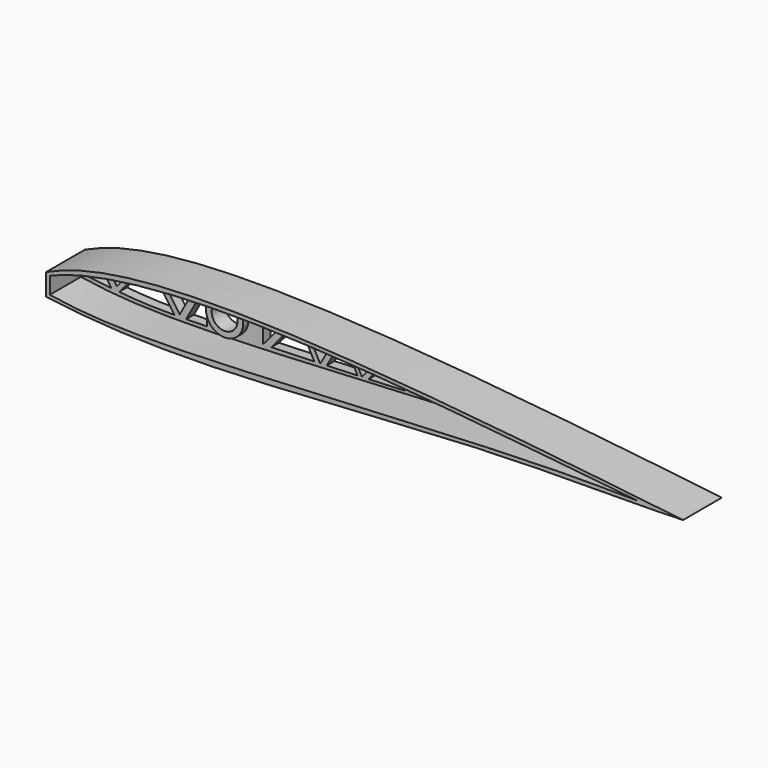
from build123d import *

# Parameters (mm, degrees)
F0_R     = 5.75
F0_R_2   = 2.5
F1_DEPTH = 3
F2_DEPTH = 15
F0_R_3   = 4
F3_DEPTH = 5


# Not quite as in the source:
# - ends of sketch curves that miss each other by under 0.0002 mm in the source are joined


with BuildPart() as f1:
    # F0 (on Front) → F1 (new body)
    with BuildSketch(Plane.XZ):
        with BuildLine():
            add(Edge.make_bspline(
                [(-96.5428803444, -1.7252441192), (-96.4749771743, -1.6951094214), (-96.406839482, -1.6654244391), (-96.3385477662, -1.6362179573)],
                knots=[0.9799990925, 0.9799990925, 0.9799990925, 0.9799990925, 1, 1, 1, 1], degree=3))
            Line((-96.5428803444, -1.7252441192), (-96.5428803444, -6.1999121678))
            add(Edge.make_bspline(
                [(-96.5428803445, -6.1999121678), (-96.1611087474, -6.2678718719), (-95.7782117135, -6.3340115071), (-95.3941463942, -6.3983665862)],
                knots=[0.0058166358, 0.0058166358, 0.0058166358, 0.0058166358, 0.0137332718, 0.0137332718, 0.0137332718, 0.0137332718], degree=3))
            Line((-95.3941463942, -6.3983665862), (-95.3941463942, -1.2117682704))
            add(Edge.make_bspline(
                [(-96.3385477662, -1.6362179573), (-96.0300606253, -1.4927727074), (-95.71523374, -1.3512900387), (-95.3941463942, -1.2117682704)],
                knots=[0, 0, 0, 0, 0.0112083174, 0.0112083174, 0.0112083174, 0.0112083174], degree=3))
        make_face()
        with BuildLine():
            Line((-95.3941463942, -1.2117682704), (-95.3941463942, -6.3983665862))
            add(Edge.make_bspline(
                [(-95.3941463942, -6.3983665862), (-80.8694306992, -8.8321693274), (-43.0853796331, -8.5556683111), (40.9195716837, -3.3120714751), (72.7341022162, -3.1550192186), (86.094097513, -3.3751911245)],
                knots=[0.0137332718, 0.0137332718, 0.0137332718, 0.0137332718, 0.3131273629, 0.7122131732, 1, 1, 1, 1], degree=3))
            add(Edge.make_bspline(
                [(-95.3941463942, -1.2117682704), (-84.6882492469, 3.4402546795), (-37.9471480513, 9.9808619504), (36.943279708, 1.696590452), (86.094097513, -3.3751911245)],
                knots=[0.0112083174, 0.0112083174, 0.0112083174, 0.0112083174, 0.384923117, 1, 1, 1, 1], degree=3))
        make_face()
        with BuildLine():
            add(Edge.make_bspline(
                [(-58.7596564737, 4.4301702308), (-57.9753522042, 4.4434334419), (-57.1958768535, 4.4485089516), (-56.4223485914, 4.4453240584)],
                knots=[0.9373807911, 0.9373807911, 0.9373807911, 0.9373807911, 1, 1, 1, 1], degree=3))
            Line((-56.4223485914, 4.4453240584), (-56.4223485914, -7.2081234653))
            add(Edge.make_bspline(
                [(-56.4223485914, -7.2081234653), (-58.5959136423, -7.2589059214), (-60.7694786933, -7.3096883775), (-62.937808184, -7.3435649348)],
                knots=[0, 0, 0, 0, 0.1686137564, 0.1686137564, 0.1686137564, 0.1686137564], degree=3))
            add(Edge.make_bspline(
                [(-62.937808184, -7.3435649348), (-64.1162804896, -7.3619766129), (-65.2932062899, -7.3753945447), (-66.4677450702, -7.3811046631)],
                knots=[0.1686137564, 0.1686137564, 0.1686137564, 0.1686137564, 0.2602541842, 0.2602541842, 0.2602541842, 0.2602541842], degree=3))
            add(Edge.make_bspline(
                [(-66.4677450702, -7.3811046631), (-69.6195281104, -7.3964273197), (-75.381287574, -7.3225727781), (-81.0300999392, -6.8840061254), (-83.592082751, -6.6398550354)],
                knots=[0.2602541842, 0.2602541842, 0.2602541842, 0.2602541842, 0.5061641117, 0.7122660034, 0.7122660034, 0.7122660034, 0.7122660034], degree=3))
            add(Edge.make_bspline(
                [(-83.592082751, -6.6398550354), (-84.4022359708, -6.5626492904), (-85.2110210526, -6.4810257561), (-86.0187478894, -6.3959850932)],
                knots=[0.7122660034, 0.7122660034, 0.7122660034, 0.7122660034, 0.7774397861, 0.7774397861, 0.7774397861, 0.7774397861], degree=3))
            add(Edge.make_bspline(
                [(-86.0187478894, -6.3959850932), (-88.7770327399, -6.1055819993), (-91.5229770142, -5.7753305369), (-94.2689212885, -5.4450790744)],
                knots=[0.7774397861, 0.7774397861, 0.7774397861, 0.7774397861, 1, 1, 1, 1], degree=3))
            Line((-94.2689212885, -5.4450790744), (-94.2689212885, -1.6795024276))
            add(Edge.make_bspline(
                [(-94.2689212885, -1.6795024276), (-92.8628953972, -1.1841994891), (-91.4581917851, -0.7250541475), (-90.0523380192, -0.2995832154)],
                knots=[0, 0, 0, 0, 0.113305349, 0.113305349, 0.113305349, 0.113305349], degree=3))
            add(Edge.make_bspline(
                [(-90.0523380192, -0.2995832154), (-89.3811327558, -0.0964480559), (-88.7096653203, 0.0990111844), (-88.0376666398, 0.2870647488)],
                knots=[0.113305349, 0.113305349, 0.113305349, 0.113305349, 0.1674014069, 0.1674014069, 0.1674014069, 0.1674014069], degree=3))
            add(Edge.make_bspline(
                [(-88.0376666398, 0.2870647488), (-84.5719605974, 1.2569154246), (-81.0921245769, 2.0297910107), (-77.561248917, 2.6427617143)],
                knots=[0.1674014069, 0.1674014069, 0.1674014069, 0.1674014069, 0.4463915894, 0.4463915894, 0.4463915894, 0.4463915894], degree=3))
            add(Edge.make_bspline(
                [(-77.561248917, 2.6427617143), (-76.8555880554, 2.7652665761), (-76.1478885806, 2.8813845552), (-75.4378558602, 2.991411566)],
                knots=[0.4463915894, 0.4463915894, 0.4463915894, 0.4463915894, 0.5021489911, 0.5021489911, 0.5021489911, 0.5021489911], degree=3))
            add(Edge.make_bspline(
                [(-75.4378558602, 2.991411566), (-74.9289069597, 3.0702785315), (-74.4187592444, 3.1460159753), (-73.9077034377, 3.2186049948)],
                knots=[0.5021489911, 0.5021489911, 0.5021489911, 0.5021489911, 0.5421156961, 0.5421156961, 0.5421156961, 0.5421156961], degree=3))
            add(Edge.make_bspline(
                [(-73.9077034377, 3.2186049948), (-73.2834974958, 3.3072655612), (-72.6579368364, 3.3912292161), (-72.0315511948, 3.4704615167)],
                knots=[0.5421156961, 0.5421156961, 0.5421156961, 0.5421156961, 0.5909312157, 0.5909312157, 0.5909312157, 0.5909312157], degree=3))
            add(Edge.make_bspline(
                [(-72.0315511948, 3.4704615167), (-67.5860174529, 4.0327826216), (-63.0989300921, 4.3567896513), (-58.7596564737, 4.4301702308)],
                knots=[0.5909312157, 0.5909312157, 0.5909312157, 0.5909312157, 0.9373807911, 0.9373807911, 0.9373807911, 0.9373807911], degree=3))
        make_face(mode=Mode.SUBTRACT)
        with Locations((-49.452, -1.371)):
            Circle(F0_R, mode=Mode.SUBTRACT)
        with BuildLine():
            Line((-39.2314642668, -6.5102223307), (-39.2314642668, 5.299675744))
            add(Edge.make_bspline(
                [(-39.2314642668, 5.299675744), (-35.9534074438, 5.1909875249), (-32.6753506208, 5.0822993057), (-29.3931825657, 4.965637255)],
                knots=[0, 0, 0, 0, 0.1482033118, 0.1482033118, 0.1482033118, 0.1482033118], degree=3))
            add(Edge.make_bspline(
                [(-29.3931825657, 4.965637255), (-28.6917369238, 4.940704928), (-27.9901035066, 4.9154084065), (-27.2882421839, 4.8896698568)],
                knots=[0.1482033118, 0.1482033118, 0.1482033118, 0.1482033118, 0.1798764515, 0.1798764515, 0.1798764515, 0.1798764515], degree=3))
            add(Edge.make_bspline(
                [(-27.2882421839, 4.8896698568), (-23.4137483209, 4.7475850185), (-19.5323092994, 4.5920298819), (-15.6371742048, 4.4099108889)],
                knots=[0.1798764515, 0.1798764515, 0.1798764515, 0.1798764515, 0.3547220816, 0.3547220816, 0.3547220816, 0.3547220816], degree=3))
            add(Edge.make_bspline(
                [(-15.6371742048, 4.4099108889), (-15.0215280405, 4.3811260441), (-14.4055397287, 4.3516775961), (-13.7891826138, 4.3215138457)],
                knots=[0.3547220816, 0.3547220816, 0.3547220816, 0.3547220816, 0.382357334, 0.382357334, 0.382357334, 0.382357334], degree=3))
            add(Edge.make_bspline(
                [(-13.7891826138, 4.3215138457), (-11.2804707946, 4.1987406107), (-7.2510801006, 3.9830392372), (-3.2013896807, 3.7279660672), (-1.676706941, 3.6272723386)],
                knots=[0.382357334, 0.382357334, 0.382357334, 0.382357334, 0.4948390149, 0.5625818971, 0.5625818971, 0.5625818971, 0.5625818971], degree=3))
            add(Edge.make_bspline(
                [(-1.676706941, 3.6272723386), (-1.1181316432, 3.5903826775), (-0.5592230256, 3.552846535), (0, 3.5147005908)],
                knots=[0.5625818971, 0.5625818971, 0.5625818971, 0.5625818971, 0.5873998474, 0.5873998474, 0.5873998474, 0.5873998474], degree=3))
            add(Edge.make_bspline(
                [(0, 3.5147005908), (3.5849822281, 3.2701603521), (7.1828854983, 3.000559448), (10.7887274401, 2.7155613037)],
                knots=[0.5873998474, 0.5873998474, 0.5873998474, 0.5873998474, 0.7464990028, 0.7464990028, 0.7464990028, 0.7464990028], degree=3))
            add(Edge.make_bspline(
                [(10.7887274401, 2.7155613037), (11.5803406425, 2.6529938652), (12.3723364586, 2.5896843385), (13.1646621709, 2.5257349704)],
                knots=[0.7464990028, 0.7464990028, 0.7464990028, 0.7464990028, 0.7814270428, 0.7814270428, 0.7814270428, 0.7814270428], degree=3))
            add(Edge.make_bspline(
                [(13.1646621709, 2.5257349704), (15.5409627422, 2.3339414724), (17.9202306891, 2.1363926795), (20.3010438532, 1.9358469013)],
                knots=[0.7814270428, 0.7814270428, 0.7814270428, 0.7814270428, 0.8861813381, 0.8861813381, 0.8861813381, 0.8861813381], degree=3))
            add(Edge.make_bspline(
                [(20.3010438532, 1.9358469013), (21.4384423664, 1.8400391019), (22.5761935461, 1.7435472975), (23.7141423287, 1.6466722377)],
                knots=[0.8861813381, 0.8861813381, 0.8861813381, 0.8861813381, 0.9362261637, 0.9362261637, 0.9362261637, 0.9362261637], degree=3))
            add(Edge.make_bspline(
                [(23.7141423287, 1.6466722377), (25.1642694588, 1.523221029), (26.6147174818, 1.3991474412), (28.0651655048, 1.2750738533)],
                knots=[0.9362261637, 0.9362261637, 0.9362261637, 0.9362261637, 1, 1, 1, 1], degree=3))
            Line((28.0651655048, 1.2750738533), (28.0651655048, -3.6732077133))
            add(Edge.make_bspline(
                [(28.0651655048, -3.6732077133), (27.4664662691, -3.7032045951), (26.8677670333, -3.7332014769), (26.269106513, -3.7631839579)],
                knots=[0, 0, 0, 0, 0.0260461999, 0.0260461999, 0.0260461999, 0.0260461999], degree=3))
            add(Edge.make_bspline(
                [(26.269106513, -3.7631839579), (23.6217461688, -3.8957706721), (20.9751429176, -4.0280757752), (18.3326447297, -4.1588539429)],
                knots=[0.0260461999, 0.0260461999, 0.0260461999, 0.0260461999, 0.1412261299, 0.1412261299, 0.1412261299, 0.1412261299], degree=3))
            add(Edge.make_bspline(
                [(18.3326447297, -4.1588539429), (17.592409558, -4.1954884427), (16.8524965153, -4.2320031222), (16.1129791965, -4.2683706067)],
                knots=[0.1412261299, 0.1412261299, 0.1412261299, 0.1412261299, 0.1734911417, 0.1734911417, 0.1734911417, 0.1734911417], degree=3))
            add(Edge.make_bspline(
                [(16.1129791965, -4.2683706067), (15.6061303016, -4.2932960802), (15.0994672951, -4.3181524099), (14.5930138711, -4.3429307826)],
                knots=[0.1734911417, 0.1734911417, 0.1734911417, 0.1734911417, 0.1956048707, 0.1956048707, 0.1956048707, 0.1956048707], degree=3))
            add(Edge.make_bspline(
                [(14.5930138711, -4.3429307826), (12.3936169659, -4.4505368792), (10.1981726621, -4.5566727509), (8.0086215303, -4.6606165755)],
                knots=[0.1956048707, 0.1956048707, 0.1956048707, 0.1956048707, 0.2916391057, 0.2916391057, 0.2916391057, 0.2916391057], degree=3))
            add(Edge.make_bspline(
                [(8.0086215303, -4.6606165755), (7.3735996711, -4.6907627547), (6.739073509, -4.7207245525), (6.105090384, -4.7504843601)],
                knots=[0.2916391057, 0.2916391057, 0.2916391057, 0.2916391057, 0.3194913159, 0.3194913159, 0.3194913159, 0.3194913159], degree=3))
            add(Edge.make_bspline(
                [(6.105090384, -4.7504843601), (5.6209562477, -4.773210105), (5.1371387803, -4.7958180605), (4.6536590632, -4.818300385)],
                knots=[0.3194913159, 0.3194913159, 0.3194913159, 0.3194913159, 0.3407603453, 0.3407603453, 0.3407603453, 0.3407603453], degree=3))
            add(Edge.make_bspline(
                [(4.6536590632, -4.818300385), (0.8798372036, -4.9937871426), (-2.8734067176, -5.1616196506), (-6.5960472566, -5.3180688061)],
                knots=[0.3407603453, 0.3407603453, 0.3407603453, 0.3407603453, 0.5067766752, 0.5067766752, 0.5067766752, 0.5067766752], degree=3))
            add(Edge.make_bspline(
                [(-6.5960472566, -5.3180688061), (-6.6322875139, -5.3195918534), (-7.325510614, -5.3487072139), (-8.0176689199, -5.3774265095), (-8.6727461513, -5.4043100041)],
                knots=[0.5067766752, 0.5067766752, 0.5067766752, 0.5067766752, 0.5083928599, 0.5376943974, 0.5376943974, 0.5376943974, 0.5376943974], degree=3))
            add(Edge.make_bspline(
                [(-8.6727461513, -5.4043100041), (-9.1152981748, -5.422471748), (-9.557439724, -5.4404808103), (-9.9991883747, -5.4583437286)],
                knots=[0.5376943974, 0.5376943974, 0.5376943974, 0.5376943974, 0.5574897042, 0.5574897042, 0.5574897042, 0.5574897042], degree=3))
            add(Edge.make_bspline(
                [(-9.9991883747, -5.4583437286), (-13.1995651312, -5.5877568424), (-16.3793198272, -5.7094992948), (-19.5451358525, -5.8260570653)],
                knots=[0.5574897042, 0.5574897042, 0.5574897042, 0.5574897042, 0.7009025691, 0.7009025691, 0.7009025691, 0.7009025691], degree=3))
            add(Edge.make_bspline(
                [(-19.5451358525, -5.8260570653), (-20.1920530868, -5.8498750098), (-20.8383882883, -5.8734764592), (-21.4841984848, -5.8968826257)],
                knots=[0.7009025691, 0.7009025691, 0.7009025691, 0.7009025691, 0.7302082057, 0.7302082057, 0.7302082057, 0.7302082057], degree=3))
            add(Edge.make_bspline(
                [(-21.4841984848, -5.8968826257), (-21.5265905055, -5.8984190441), (-21.568980264, -5.8999546211), (-21.6113677766, -5.9014893627)],
                knots=[0.7302082057, 0.7302082057, 0.7302082057, 0.7302082057, 0.7321318749, 0.7321318749, 0.7321318749, 0.7321318749], degree=3))
            add(Edge.make_bspline(
                [(-21.6113677766, -5.9014893627), (-22.2032423382, -5.9229196008), (-22.7946789769, -5.9441869474), (-23.3857216062, -5.9653077367)],
                knots=[0.7321318749, 0.7321318749, 0.7321318749, 0.7321318749, 0.7589928716, 0.7589928716, 0.7589928716, 0.7589928716], degree=3))
            add(Edge.make_bspline(
                [(-23.3857216062, -5.9653077367), (-27.8246304727, -6.1239312512), (-32.2413153798, -6.2742882557), (-36.6543788181, -6.4232982046)],
                knots=[0.7589928716, 0.7589928716, 0.7589928716, 0.7589928716, 0.9607270796, 0.9607270796, 0.9607270796, 0.9607270796], degree=3))
            add(Edge.make_bspline(
                [(-36.6543788181, -6.4232982046), (-37.5134988009, -6.452306948), (-38.3724815339, -6.4812646393), (-39.2314642668, -6.5102223307)],
                knots=[0.9607270796, 0.9607270796, 0.9607270796, 0.9607270796, 1, 1, 1, 1], degree=3))
        make_face(mode=Mode.SUBTRACT)
        with Locations((33.779, -1.031)):
            Circle(F0_R_2, mode=Mode.SUBTRACT)
        with BuildLine():
            Line((-62.937808184, -7.3435649348), (-56.4223485914, 4.4453240584))
            add(Edge.make_bspline(
                [(-58.7596564737, 4.4301702308), (-57.9753522042, 4.4434334419), (-57.1958768535, 4.4485089516), (-56.4223485914, 4.4453240584)],
                knots=[0.9373807911, 0.9373807911, 0.9373807911, 0.9373807911, 1, 1, 1, 1], degree=3))
            Line((-58.7596564737, 4.4301702308), (-64.903050668, -6.6855141148))
            Line((-64.903050668, -6.6855141148), (-72.0315511948, 3.4704615167))
            add(Edge.make_bspline(
                [(-73.9077034377, 3.2186049948), (-73.2834974958, 3.3072655612), (-72.6579368364, 3.3912292161), (-72.0315511948, 3.4704615167)],
                knots=[0.5421156961, 0.5421156961, 0.5421156961, 0.5421156961, 0.5909312157, 0.5909312157, 0.5909312157, 0.5909312157], degree=3))
            Line((-73.9077034377, 3.2186049948), (-66.4677450702, -7.3811046631))
            add(Edge.make_bspline(
                [(-62.937808184, -7.3435649348), (-64.1162804896, -7.3619766129), (-65.2932062899, -7.3753945447), (-66.4677450702, -7.3811046631)],
                knots=[0.1686137564, 0.1686137564, 0.1686137564, 0.1686137564, 0.2602541842, 0.2602541842, 0.2602541842, 0.2602541842], degree=3))
        make_face()
        with BuildLine():
            add(Edge.make_bspline(
                [(-83.592082751, -6.6398550354), (-84.4022359708, -6.5626492904), (-85.2110210526, -6.4810257561), (-86.0187478894, -6.3959850932)],
                knots=[0.7122660034, 0.7122660034, 0.7122660034, 0.7122660034, 0.7774397861, 0.7774397861, 0.7774397861, 0.7774397861], degree=3))
            Line((-83.592082751, -6.6398550354), (-75.4378558602, 2.991411566))
            add(Edge.make_bspline(
                [(-77.561248917, 2.6427617143), (-76.8555880554, 2.7652665761), (-76.1478885806, 2.8813845552), (-75.4378558602, 2.991411566)],
                knots=[0.4463915894, 0.4463915894, 0.4463915894, 0.4463915894, 0.5021489911, 0.5021489911, 0.5021489911, 0.5021489911], degree=3))
            Line((-77.561248917, 2.6427617143), (-84.3168773909, -5.3365672599))
            Line((-84.3168773909, -5.3365672599), (-88.0376666398, 0.2870647488))
            add(Edge.make_bspline(
                [(-90.0523380192, -0.2995832154), (-89.3811327558, -0.0964480559), (-88.7096653203, 0.0990111844), (-88.0376666398, 0.2870647488)],
                knots=[0.113305349, 0.113305349, 0.113305349, 0.113305349, 0.1674014069, 0.1674014069, 0.1674014069, 0.1674014069], degree=3))
            Line((-90.0523380192, -0.2995832154), (-86.0187478894, -6.3959850932))
        make_face()
        with BuildLine():
            Line((-29.3931825657, 4.965637255), (-39.2314642668, -6.5102223307))
            add(Edge.make_bspline(
                [(-36.6543788181, -6.4232982046), (-37.5134988009, -6.452306948), (-38.3724815339, -6.4812646393), (-39.2314642668, -6.5102223307)],
                knots=[0.9607270796, 0.9607270796, 0.9607270796, 0.9607270796, 1, 1, 1, 1], degree=3))
            Line((-36.6543788181, -6.4232982046), (-28.2822091366, 3.3424156275))
            Line((-28.2822091366, 3.3424156275), (-23.3857216062, -5.9653077367))
            add(Edge.make_bspline(
                [(-21.6113677766, -5.9014893627), (-22.2032423382, -5.9229196008), (-22.7946789769, -5.9441869474), (-23.3857216062, -5.9653077367)],
                knots=[0.7321318749, 0.7321318749, 0.7321318749, 0.7321318749, 0.7589928716, 0.7589928716, 0.7589928716, 0.7589928716], degree=3))
            Line((-21.6113677766, -5.9014893627), (-27.2882421839, 4.8896698568))
            add(Edge.make_bspline(
                [(-29.3931825657, 4.965637255), (-28.6917369238, 4.940704928), (-27.9901035066, 4.9154084065), (-27.2882421839, 4.8896698568)],
                knots=[0.1482033118, 0.1482033118, 0.1482033118, 0.1482033118, 0.1798764515, 0.1798764515, 0.1798764515, 0.1798764515], degree=3))
        make_face()
        with BuildLine():
            add(Edge.make_bspline(
                [(-15.6371742048, 4.4099108889), (-15.0215280405, 4.3811260441), (-14.4055397287, 4.3516775961), (-13.7891826138, 4.3215138457)],
                knots=[0.3547220816, 0.3547220816, 0.3547220816, 0.3547220816, 0.382357334, 0.382357334, 0.382357334, 0.382357334], degree=3))
            Line((-15.6371742048, 4.4099108889), (-21.4841984848, -5.8968826257))
            add(Edge.make_bspline(
                [(-19.5451358525, -5.8260570653), (-20.1920530868, -5.8498750098), (-20.8383882883, -5.8734764592), (-21.4841984848, -5.8968826257)],
                knots=[0.7009025691, 0.7009025691, 0.7009025691, 0.7009025691, 0.7302082057, 0.7302082057, 0.7302082057, 0.7302082057], degree=3))
            Line((-19.5451358525, -5.8260570653), (-14.4918043747, 3.0816610505))
            Line((-14.4918043747, 3.0816610505), (-9.9991883747, -5.4583437286))
            add(Edge.make_bspline(
                [(-8.6727461513, -5.4043100041), (-9.1152981748, -5.422471748), (-9.557439724, -5.4404808103), (-9.9991883747, -5.4583437286)],
                knots=[0.5376943974, 0.5376943974, 0.5376943974, 0.5376943974, 0.5574897042, 0.5574897042, 0.5574897042, 0.5574897042], degree=3))
            Line((-8.6727461513, -5.4043100041), (-13.7891826138, 4.3215138457))
        make_face()
        with BuildLine():
            add(Edge.make_bspline(
                [(-1.676706941, 3.6272723386), (-1.1181316432, 3.5903826775), (-0.5592230256, 3.552846535), (0, 3.5147005908)],
                knots=[0.5625818971, 0.5625818971, 0.5625818971, 0.5625818971, 0.5873998474, 0.5873998474, 0.5873998474, 0.5873998474], degree=3))
            Line((-1.676706941, 3.6272723386), (-8.6727461513, -5.4043100041))
            add(Edge.make_bspline(
                [(-6.5960472566, -5.3180688061), (-6.6322875139, -5.3195918534), (-7.325510614, -5.3487072139), (-8.0176689199, -5.3774265095), (-8.6727461513, -5.4043100041)],
                knots=[0.5067766752, 0.5067766752, 0.5067766752, 0.5067766752, 0.5083928599, 0.5376943974, 0.5376943974, 0.5376943974, 0.5376943974], degree=3))
            Line((-6.5960472566, -5.3180688061), (-0.6485358524, 2.3599097423))
            Line((-0.6485358524, 2.3599097423), (4.6536590632, -4.818300385))
            add(Edge.make_bspline(
                [(6.105090384, -4.7504843601), (5.6209562477, -4.773210105), (5.1371387803, -4.7958180605), (4.6536590632, -4.818300385)],
                knots=[0.3194913159, 0.3194913159, 0.3194913159, 0.3194913159, 0.3407603453, 0.3407603453, 0.3407603453, 0.3407603453], degree=3))
            Line((6.105090384, -4.7504843601), (0, 3.5147005908))
        make_face()
        with BuildLine():
            add(Edge.make_bspline(
                [(10.7887274401, 2.7155613037), (11.5803406425, 2.6529938652), (12.3723364586, 2.5896843385), (13.1646621709, 2.5257349704)],
                knots=[0.7464990028, 0.7464990028, 0.7464990028, 0.7464990028, 0.7814270428, 0.7814270428, 0.7814270428, 0.7814270428], degree=3))
            Line((10.7887274401, 2.7155613037), (6.105090384, -4.7504843601))
            add(Edge.make_bspline(
                [(8.0086215303, -4.6606165755), (7.3735996711, -4.6907627547), (6.739073509, -4.7207245525), (6.105090384, -4.7504843601)],
                knots=[0.2916391057, 0.2916391057, 0.2916391057, 0.2916391057, 0.3194913159, 0.3194913159, 0.3194913159, 0.3194913159], degree=3))
            Line((8.0086215303, -4.6606165755), (11.9821707942, 1.6734993897))
            Line((11.9821707942, 1.6734993897), (14.5930138711, -4.3429307826))
            add(Edge.make_bspline(
                [(16.1129791965, -4.2683706067), (15.6061303016, -4.2932960802), (15.0994672951, -4.3181524099), (14.5930138711, -4.3429307826)],
                knots=[0.1734911417, 0.1734911417, 0.1734911417, 0.1734911417, 0.1956048707, 0.1956048707, 0.1956048707, 0.1956048707], degree=3))
            Line((16.1129791965, -4.2683706067), (13.1646621709, 2.5257349704))
        make_face()
        with BuildLine():
            add(Edge.make_bspline(
                [(20.3010438532, 1.9358469013), (21.4384423664, 1.8400391019), (22.5761935461, 1.7435472975), (23.7141423287, 1.6466722377)],
                knots=[0.8861813381, 0.8861813381, 0.8861813381, 0.8861813381, 0.9362261637, 0.9362261637, 0.9362261637, 0.9362261637], degree=3))
            Line((20.3010438532, 1.9358469013), (16.1129791965, -4.2683706067))
            add(Edge.make_bspline(
                [(18.3326447297, -4.1588539429), (17.592409558, -4.1954884427), (16.8524965153, -4.2320031222), (16.1129791965, -4.2683706067)],
                knots=[0.1412261299, 0.1412261299, 0.1412261299, 0.1412261299, 0.1734911417, 0.1734911417, 0.1734911417, 0.1734911417], degree=3))
            Line((18.3326447297, -4.1588539429), (22.0675114827, 1.3739941859))
            Line((22.0675114827, 1.3739941859), (26.269106513, -3.7631839579))
            add(Edge.make_bspline(
                [(28.0651655048, -3.6732077133), (27.4664662691, -3.7032045951), (26.8677670333, -3.7332014769), (26.269106513, -3.7631839579)],
                knots=[0, 0, 0, 0, 0.0260461999, 0.0260461999, 0.0260461999, 0.0260461999], degree=3))
            Line((28.0651655048, -3.6732077133), (23.7141423287, 1.6466722377))
        make_face()
    extrude(amount=F1_DEPTH)

    # F0 (on Front) → F2 (join)
    with BuildSketch(Plane.XZ):
        with BuildLine():
            add(Edge.make_bspline(
                [(-96.5428803444, -0.598909816), (-84.374379176, 5.1984880484), (-38.2751930486, 10.925719155), (42.6881882799, 2.4723259958), (100, -4.047003109)],
                knots=[0.0044628662, 0.0044628662, 0.0044628662, 0.0044628662, 0.374886421, 1, 1, 1, 1], degree=3))
            Line((-96.5428803444, -0.598909816), (-96.5428803444, -1.7252441192))
            add(Edge.make_bspline(
                [(-96.5428803444, -1.7252441192), (-96.4749771743, -1.6951094214), (-96.406839482, -1.6654244391), (-96.3385477662, -1.6362179573)],
                knots=[0.9799990925, 0.9799990925, 0.9799990925, 0.9799990925, 1, 1, 1, 1], degree=3))
            add(Edge.make_bspline(
                [(-96.3385477662, -1.6362179573), (-96.0300606253, -1.4927727074), (-95.71523374, -1.3512900387), (-95.3941463942, -1.2117682704)],
                knots=[0, 0, 0, 0, 0.0112083174, 0.0112083174, 0.0112083174, 0.0112083174], degree=3))
            add(Edge.make_bspline(
                [(-95.3941463942, -1.2117682704), (-84.6882492469, 3.4402546795), (-37.9471480513, 9.9808619504), (36.943279708, 1.696590452), (86.094097513, -3.3751911245)],
                knots=[0.0112083174, 0.0112083174, 0.0112083174, 0.0112083174, 0.384923117, 1, 1, 1, 1], degree=3))
            add(Edge.make_bspline(
                [(-95.3941463942, -6.3983665862), (-80.8694306992, -8.8321693274), (-43.0853796331, -8.5556683111), (40.9195716837, -3.3120714751), (72.7341022162, -3.1550192186), (86.094097513, -3.3751911245)],
                knots=[0.0137332718, 0.0137332718, 0.0137332718, 0.0137332718, 0.3131273629, 0.7122131732, 1, 1, 1, 1], degree=3))
            add(Edge.make_bspline(
                [(-96.5428803445, -6.1999121678), (-96.1611087474, -6.2678718719), (-95.7782117135, -6.3340115071), (-95.3941463942, -6.3983665862)],
                knots=[0.0058166358, 0.0058166358, 0.0058166358, 0.0058166358, 0.0137332718, 0.0137332718, 0.0137332718, 0.0137332718], degree=3))
            Line((-96.5428803445, -6.1999121678), (-96.5428803444, -7.3406707446))
            add(Edge.make_bspline(
                [(-96.5428803444, -7.3406707446), (-80.7020161693, -9.4302402111), (-44.2471235075, -11.1181020976), (41.8622965332, -3.5518856086), (82.0915186506, -4.6802794425), (100, -4.047003109)],
                knots=[0, 0, 0, 0, 0.2987594418, 0.6837410955, 1, 1, 1, 1], degree=3))
        make_face()
        with BuildLine():
            add(Edge.make_bspline(
                [(-96.5428803444, -1.7252441192), (-96.4749771743, -1.6951094214), (-96.406839482, -1.6654244391), (-96.3385477662, -1.6362179573)],
                knots=[0.9799990925, 0.9799990925, 0.9799990925, 0.9799990925, 1, 1, 1, 1], degree=3))
            Line((-96.5428803444, -1.7252441192), (-96.5428803444, -6.1999121678))
            add(Edge.make_bspline(
                [(-96.5428803445, -6.1999121678), (-96.1611087474, -6.2678718719), (-95.7782117135, -6.3340115071), (-95.3941463942, -6.3983665862)],
                knots=[0.0058166358, 0.0058166358, 0.0058166358, 0.0058166358, 0.0137332718, 0.0137332718, 0.0137332718, 0.0137332718], degree=3))
            Line((-95.3941463942, -6.3983665862), (-95.3941463942, -1.2117682704))
            add(Edge.make_bspline(
                [(-96.3385477662, -1.6362179573), (-96.0300606253, -1.4927727074), (-95.71523374, -1.3512900387), (-95.3941463942, -1.2117682704)],
                knots=[0, 0, 0, 0, 0.0112083174, 0.0112083174, 0.0112083174, 0.0112083174], degree=3))
        make_face()
    extrude(amount=F2_DEPTH)

    # F0 (on Front) → F3 (join)
    with BuildSketch(Plane.XZ):
        with Locations((-49.452, -1.371)):
            Circle(F0_R)
        with Locations((-49.452, -1.371)):
            Circle(F0_R_3, mode=Mode.SUBTRACT)
    extrude(amount=F3_DEPTH)


solid = f1.part
